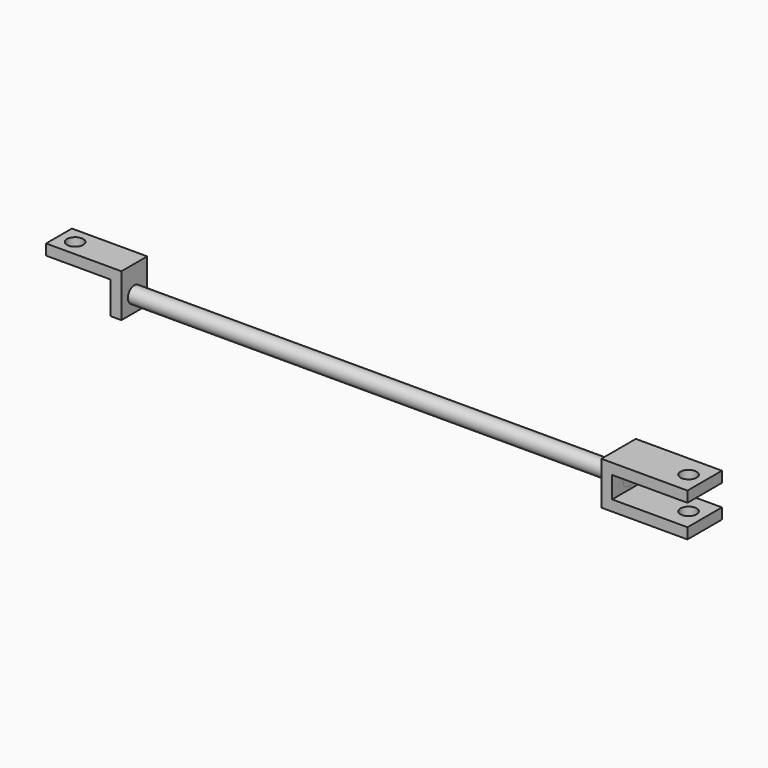
from build123d import *

# Parameters (mm, degrees)
F0_R      = 4.7625
F1_DEPTH  = 298.45
F3_DEPTH  = 9.525
F5_R      = 4.7625
F6_DEPTH  = 25.401
F8_DEPTH  = 12.7
F10_R     = 4.7625
F11_DEPTH = 25.401


# Not quite as in the source:
# - a length typed as a fraction of an inch, garbled in the dataset ("3 / 203.2 mm" for 3/8 in), is restored


with BuildPart() as f1:
    # F0 (on Right) → F1 (new body)
    with BuildSketch(Plane.YZ):
        Circle(F0_R)
    extrude(amount=F1_DEPTH)


with BuildPart() as f3:
    # F2 (on Front) → F3 (new body, symmetric)
    with BuildSketch(Plane.XZ):
        Polygon((-38.1, 9.525), (0, 9.525), (0, -9.525), (6.35, -9.525), (6.35, 15.875), (-38.1, 15.875), align=None)
    extrude(amount=F3_DEPTH, both=True)

    # F4: cut F1
    add(f1.part, mode=Mode.SUBTRACT)

    # F5 (on face) → F6 (cut, through all)
    with BuildSketch(Plane.XY.offset(15.875)):
        with Locations((-28.575, 0)):
            Circle(F5_R)
    extrude(amount=-F6_DEPTH, mode=Mode.SUBTRACT)


with BuildPart() as f8:
    # F7 (on Front) → F8 (new body, symmetric)
    with BuildSketch(Plane.XZ):
        Polygon((342.9, 12.7), (292.1, 12.7), (292.1, -12.7), (342.9, -12.7), (342.9, -6.35), (298.45, -6.35), (298.45, 6.35), (342.9, 6.35), align=None)
    extrude(amount=F8_DEPTH, both=True)

    # F9: cut F1
    add(f1.part, mode=Mode.SUBTRACT)

    # F10 (on face) → F11 (cut, through all)
    with BuildSketch(Plane.XY.offset(12.7)):
        with Locations((333.375, 0)):
            Circle(F10_R)
    extrude(amount=-F11_DEPTH, mode=Mode.SUBTRACT)


solid = Compound([f1.part, f3.part, f8.part])
